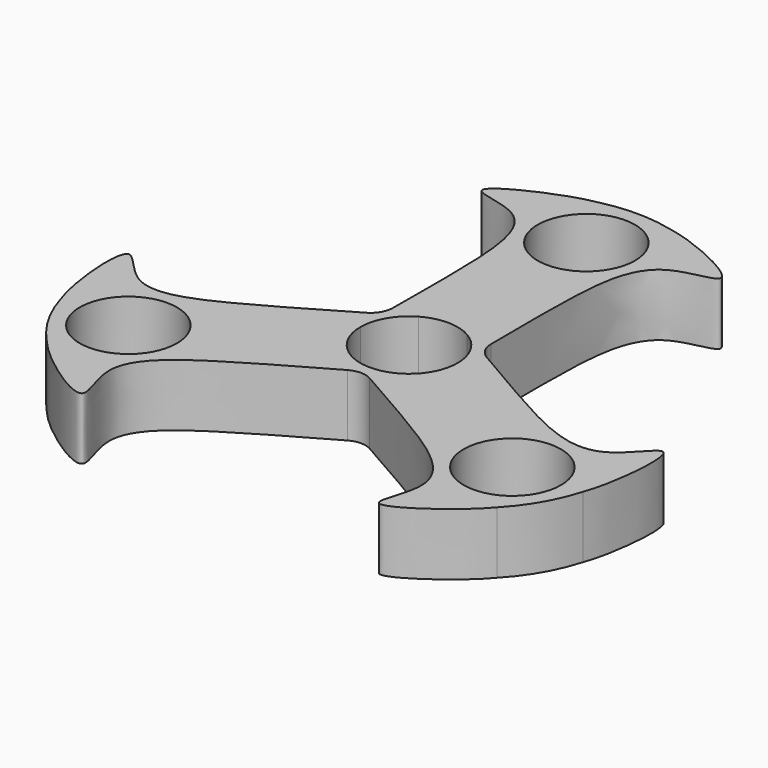
from build123d import *

# Parameters (mm, degrees)
F0_R     = 10.9601
F1_DEPTH = 13.97


# Not quite as in the source:
# - ends of sketch curves that miss each other by under 0.0002 mm in the source are joined


with BuildPart() as f1:
    # F0 (on Top) → F1 (new body)
    with BuildSketch(Plane.XY):
        with BuildLine():
            add(Edge.make_bspline(
                [(-11.0406858774, 9.2820621436), (-11.0076014857, 15.9358459435), (-10.7449299367, 33.6582046386), (-12.7235225678, 52.8517669252), (-35.2698533951, 52.5635012401), (-14.5511130353, 62.1315011674), (-8.1170605379, 63.1931111653)],
                knots=[0.1081445238, 0.1081445238, 0.1081445238, 0.1081445238, 0.3115819068, 0.5662847157, 0.7446706117, 1, 1, 1, 1], degree=3))
            add(Edge.make_bspline(
                [(-11.0485298495, 6.3788758502), (-11.0487262833, 7.3148332558), (-11.0456445743, 8.2847913468), (-11.0406858774, 9.2820621436)],
                knots=[0.0776532775, 0.0776532775, 0.0776532775, 0.0776532775, 0.1081445238, 0.1081445238, 0.1081445238, 0.1081445238], degree=3))
            add(Edge.make_bspline(
                [(-5.490177696, 9.4858849998), (-7.1072740945, 8.6285327965), (-8.9879537059, 7.5678930589), (-11.0485298495, 6.3788758502)],
                knots=[0, 0, 0, 0, 0.077526237, 0.077526237, 0.077526237, 0.077526237], degree=3))
            ThreePointArc((-5.490177696, 9.4858849998), (-0.0040332803, 10.9600992579), (5.4831884226, 9.4899123669))
            add(Edge.make_bspline(
                [(5.4831884226, 9.4899123669), (7.1021143759, 8.6315901702), (8.9852286388, 7.5695155183), (11.0485570412, 6.378854666)],
                knots=[0, 0, 0, 0, 0.0776139489, 0.0776139489, 0.0776139489, 0.0776139489], degree=3))
            add(Edge.make_bspline(
                [(11.0485570412, 6.378854666), (11.0487264298, 7.3147693284), (11.0456448051, 8.2847324252), (11.0406861431, 9.2820087008)],
                knots=[0.0776525355, 0.0776525355, 0.0776525355, 0.0776525355, 0.1081439792, 0.1081439792, 0.1081439792, 0.1081439792], degree=3))
            add(Edge.make_bspline(
                [(11.0406861431, 9.2820087008), (11.0076021103, 15.9358038046), (10.7449282436, 33.658188215), (12.7235225678, 52.8517669252), (35.2698533951, 52.5635012401), (14.5511130353, 62.1315011674), (8.1170605379, 63.1931111653)],
                knots=[0.1081439792, 0.1081439792, 0.1081439792, 0.1081439792, 0.3115819068, 0.5662847157, 0.7446706117, 1, 1, 1, 1], degree=3))
            ThreePointArc((8.1170605379, 63.1931111653), (0, 64.1708099603), (-8.1170605379, 63.1931111653))
        make_face()
        with Locations((0, 49.9257668853)):
            Circle(F0_R, mode=Mode.SUBTRACT)
        with BuildLine():
            add(Edge.make_bspline(
                [(-11.0485298495, 6.3788758502), (-11.0487262833, 7.3148332558), (-11.0456445743, 8.2847913468), (-11.0406858774, 9.2820621436)],
                knots=[0.0776532775, 0.0776532775, 0.0776532775, 0.0776532775, 0.1081445238, 0.1081445238, 0.1081445238, 0.1081445238], degree=3))
            ThreePointArc((-11.0406858774, 9.2820621436), (-11.7212314541, 6.7672907696), (-13.5588398975, 4.9205605363))
            add(Edge.make_bspline(
                [(-11.0485298494, 6.3788758502), (-11.8591570463, 5.9111184756), (-12.6976254335, 5.423493116), (-13.5588398975, 4.9205605363)],
                knots=[0.077526237, 0.077526237, 0.077526237, 0.077526237, 0.1080249286, 0.1080249286, 0.1080249286, 0.1080249286], degree=3))
        make_face()
        with BuildLine():
            add(Edge.make_bspline(
                [(-5.490177696, 9.4858849998), (-7.1072740945, 8.6285327965), (-8.9879537059, 7.5678930589), (-11.0485298494, 6.3788758502)],
                knots=[0, 0, 0, 0, 0.077526237, 0.077526237, 0.077526237, 0.077526237], degree=3))
            add(Edge.make_bspline(
                [(-10.9601, 0), (-11.0262676612, 1.8321200044), (-11.0480295836, 3.9952356637), (-11.0485298494, 6.3788758502)],
                knots=[0, 0, 0, 0, 0.0776532775, 0.0776532775, 0.0776532775, 0.0776532775], degree=3))
            ThreePointArc((-10.9601, 0), (-9.4946463892, 5.4749869364), (-5.490177696, 9.4858849998))
        make_face()
        with BuildLine():
            add(Edge.make_bspline(
                [(-10.9601, 0), (-11.0262676612, 1.8321200044), (-11.0480295836, 3.9952356637), (-11.0485298495, 6.3788758502)],
                knots=[0, 0, 0, 0, 0.0776532775, 0.0776532775, 0.0776532775, 0.0776532775], degree=3))
            add(Edge.make_bspline(
                [(-11.0485298494, 6.3788758502), (-11.8591570463, 5.9111184756), (-12.6976254335, 5.423493116), (-13.5588398975, 4.9205605363)],
                knots=[0.077526237, 0.077526237, 0.077526237, 0.077526237, 0.1080249286, 0.1080249286, 0.1080249286, 0.1080249286], degree=3))
            add(Edge.make_bspline(
                [(-13.5588398975, 4.9205605363), (-19.3068312047, 1.5638448547), (-34.5281439644, -7.528078893), (-52.142861772, -15.4128297215), (-63.1663817793, 4.2569983796), (-61.0931425999, -18.46995707), (-58.7954975783, -24.572814981)],
                knots=[0.1080249286, 0.1080249286, 0.1080249286, 0.1080249286, 0.3115819068, 0.5662847157, 0.7446706117, 1, 1, 1, 1], degree=3))
            ThreePointArc((-58.7954975783, -24.572814981), (-55.5748737612, -32.0861611265), (-50.6784370404, -38.6319762408))
            add(Edge.make_bspline(
                [(-2.5181212243, -14.2025838003), (-8.299112665, -17.5021291831), (-23.7835931212, -26.1382048835), (-39.4193392042, -37.4506172602), (-27.8965283843, -56.8321796762), (-46.5420295646, -43.6732241539), (-50.6784370404, -38.6319762408)],
                knots=[0.1080252275, 0.1080252275, 0.1080252275, 0.1080252275, 0.3115819068, 0.5662847157, 0.7446706117, 1, 1, 1, 1], degree=3))
            add(Edge.make_bspline(
                [(-7.2729e-06, -12.7577373339), (-0.8104171528, -13.2258861395), (-1.6519542861, -13.7082123502), (-2.5181212243, -14.2025838003)],
                knots=[0.0775262953, 0.0775262953, 0.0775262953, 0.0775262953, 0.1080252275, 0.1080252275, 0.1080252275, 0.1080252275], degree=3))
            add(Edge.make_bspline(
                [(-5.4765933563, -9.4937198832), (-3.9238847553, -10.4665376582), (-2.0626684707, -11.5662545114), (-7.2729e-06, -12.7577373338)],
                knots=[0, 0, 0, 0, 0.0776097901, 0.0776097901, 0.0776097901, 0.0776097901], degree=3))
            ThreePointArc((-5.4765933563, -9.4937198832), (-9.4907271285, -5.4817780494), (-10.9601, 0))
        make_face()
        with Locations((-43.2471101221, -24.9687234709)):
            Circle(F0_R, mode=Mode.SUBTRACT)
        with BuildLine():
            ThreePointArc((13.5587994149, 4.920530574), (11.7212198447, 6.7672575808), (11.0406861431, 9.2820087008))
            add(Edge.make_bspline(
                [(11.0485298351, 6.3788075199), (11.0487264298, 7.3147693284), (11.0456448051, 8.2847324252), (11.0406861431, 9.2820087008)],
                knots=[0.0776525355, 0.0776525355, 0.0776525355, 0.0776525355, 0.1081439792, 0.1081439792, 0.1081439792, 0.1081439792], degree=3))
            Line((11.0485298351, 6.3788075199), (11.052011444, 6.3768612511))
            add(Edge.make_bspline(
                [(11.052011444, 6.3768612511), (11.8615676965, 5.9096893035), (12.698853869, 5.4227328428), (13.5587994149, 4.920530574)],
                knots=[0.0776572602, 0.0776572602, 0.0776572602, 0.0776572602, 0.1081064771, 0.1081064771, 0.1081064771, 0.1081064771], degree=3))
        make_face()
        with BuildLine():
            ThreePointArc((5.469922304, -9.4975650563), (-0.0038499446, -10.9600993238), (-5.4765933563, -9.4937198832))
            add(Edge.make_bspline(
                [(-5.4765933563, -9.4937198832), (-3.9238847553, -10.4665376582), (-2.0626684707, -11.5662545114), (-7.2729e-06, -12.7577373338)],
                knots=[0, 0, 0, 0, 0.0776097901, 0.0776097901, 0.0776097901, 0.0776097901], degree=3))
            add(Edge.make_bspline(
                [(5.469922304, -9.4975650563), (3.9188841505, -10.4693362468), (2.0600017585, -11.567733619), (-7.2729e-06, -12.7577373339)],
                knots=[0, 0, 0, 0, 0.0775262953, 0.0775262953, 0.0775262953, 0.0775262953], degree=3))
        make_face()
        with BuildLine():
            add(Edge.make_bspline(
                [(5.4831884226, 9.4899123669), (7.1021143759, 8.6315901702), (8.9852286388, 7.5695155183), (11.0485570412, 6.378854666)],
                knots=[0, 0, 0, 0, 0.0776139489, 0.0776139489, 0.0776139489, 0.0776139489], degree=3))
            ThreePointArc((5.4831884226, 9.4899123669), (9.4926309694, 5.478480564), (10.9601, 0))
            add(Edge.make_bspline(
                [(10.9601, 0), (11.026267029, 1.8321024976), (11.0480291677, 3.9951943245), (11.0485570412, 6.378854666)],
                knots=[0, 0, 0, 0, 0.0776525355, 0.0776525355, 0.0776525355, 0.0776525355], degree=3))
        make_face()
        with BuildLine():
            Line((11.052011444, 6.3768612511), (11.0485298351, 6.3788075199))
            add(Edge.make_bspline(
                [(10.9601, 0), (11.026267029, 1.8321024976), (11.0480291677, 3.9951943245), (11.0485298351, 6.3788075199)],
                knots=[0, 0, 0, 0, 0.0776525355, 0.0776525355, 0.0776525355, 0.0776525355], degree=3))
            ThreePointArc((10.9601, 0), (9.4888009636, -5.4851115105), (5.469922304, -9.4975650563))
            add(Edge.make_bspline(
                [(5.469922304, -9.4975650563), (3.9188841505, -10.4693362468), (2.0600017585, -11.567733619), (-7.2729e-06, -12.7577373339)],
                knots=[0, 0, 0, 0, 0.0775262953, 0.0775262953, 0.0775262953, 0.0775262953], degree=3))
            add(Edge.make_bspline(
                [(-7.2729e-06, -12.7577373338), (0.8104429093, -13.2258886093), (1.6519925735, -13.7082069048), (2.5181473988, -14.2025610809)],
                knots=[0.0776097901, 0.0776097901, 0.0776097901, 0.0776097901, 0.1081038279, 0.1081038279, 0.1081038279, 0.1081038279], degree=3))
            add(Edge.make_bspline(
                [(2.5181473988, -14.2025610809), (8.2977532688, -17.5012465062), (23.7788524629, -26.1357563444), (39.4126681519, -37.4467720871), (27.889857332, -56.8283345031), (46.5353585123, -43.6693789807), (50.6717659881, -38.6281310677)],
                knots=[0.1081038279, 0.1081038279, 0.1081038279, 0.1081038279, 0.3115819068, 0.5662847157, 0.7446706117, 1, 1, 1, 1], degree=3))
            ThreePointArc((50.6717659881, -38.6281310677), (55.5851230712, -32.092084929), (58.788826526, -24.5689698079))
            add(Edge.make_bspline(
                [(13.5587994149, 4.920530574), (19.3053801646, 1.5645670436), (34.5237357223, -7.5252510333), (52.1361800766, -15.4089802612), (63.1597156942, 4.26084514), (61.0864673005, -18.4661231778), (58.788826526, -24.5689698079)],
                knots=[0.1081064771, 0.1081064771, 0.1081064771, 0.1081064771, 0.3115831793, 0.5662855174, 0.7446710837, 1, 1, 1, 1], degree=3))
            add(Edge.make_bspline(
                [(11.052011444, 6.3768612511), (11.8615676965, 5.9096893035), (12.698853869, 5.4227328428), (13.5587994149, 4.920530574)],
                knots=[0.0776572602, 0.0776572602, 0.0776572602, 0.0776572602, 0.1081064771, 0.1081064771, 0.1081064771, 0.1081064771], degree=3))
        make_face()
        with Locations((43.2404390698, -24.9648782978)):
            Circle(F0_R, mode=Mode.SUBTRACT)
        with BuildLine():
            add(Edge.make_bspline(
                [(-7.2729e-06, -12.7577373338), (0.8104429093, -13.2258886093), (1.6519925735, -13.7082069048), (2.5181473988, -14.2025610809)],
                knots=[0.0776097901, 0.0776097901, 0.0776097901, 0.0776097901, 0.1081038279, 0.1081038279, 0.1081038279, 0.1081038279], degree=3))
            add(Edge.make_bspline(
                [(-7.2729e-06, -12.7577373339), (-0.8104171528, -13.2258861395), (-1.6519542861, -13.7082123502), (-2.5181212243, -14.2025838003)],
                knots=[0.0775262953, 0.0775262953, 0.0775262953, 0.0775262953, 0.1080252275, 0.1080252275, 0.1080252275, 0.1080252275], degree=3))
            ThreePointArc((-2.5181212243, -14.2025838003), (1.00736e-05, -13.5345334093), (2.5181473988, -14.2025610809))
        make_face()
    extrude(amount=F1_DEPTH)


solid = f1.part
